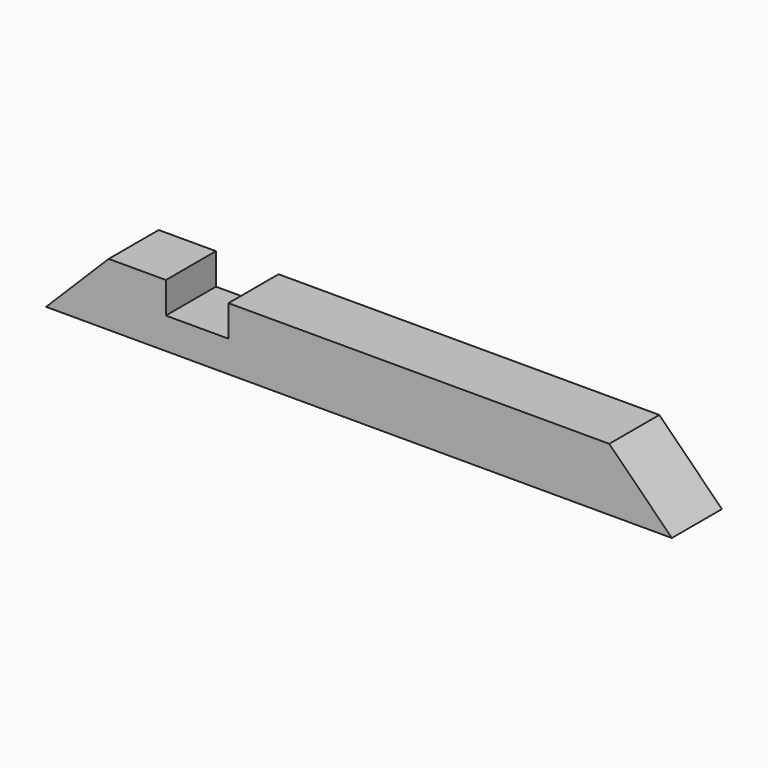
from build123d import *

# Parameters (mm, degrees)
F0_W     = 254
F0_H     = 25.4
F1_DEPTH = 25.4
F2_SIZE2 = 25.39999
F2_SIZE  = 25.39999
F3_SIZE2 = 25.39999
F3_SIZE  = 25.39999
F4_W     = 25.4
F4_H     = 25.4
F5_DEPTH = 12.7


# Not quite as in the source:
# - a fillet or chamfer is up to 0.001 mm smaller than in the source, because OpenCascade refuses the exact size


with BuildPart() as f1:
    # F0 (on Front) → F1 (new body)
    with BuildSketch(Plane.XZ):
        with Locations((52.2324490321, -35.310111469)):
            Rectangle(F0_W, F0_H)
    extrude(amount=-F1_DEPTH)

    # F2 (size 25.4 and 25.4 in the source; OpenCascade refuses exactly that, so slightly less here)
    f2_edges = [f1.edges().sort_by_distance(p)[0] for p in [
        (179.232449, 12.7, -22.610111),
    ]]
    chamfer(f2_edges, length=F2_SIZE, length2=F2_SIZE2)

    # F3 (size 25.4 and 25.4 in the source; OpenCascade refuses exactly that, so slightly less here)
    f3_edges = [f1.edges().sort_by_distance(p)[0] for p in [
        (-74.767551, 12.7, -22.610111),
    ]]
    chamfer(f3_edges, length=F3_SIZE, length2=F3_SIZE2)

    # F4 (on face) → F5 (cut)
    with BuildSketch(Plane.XY.offset(-22.610111469)):
        with Locations((-13.4418782175, 12.7)):
            Rectangle(F4_W, F4_H)
    extrude(amount=-F5_DEPTH, mode=Mode.SUBTRACT)


solid = f1.part
